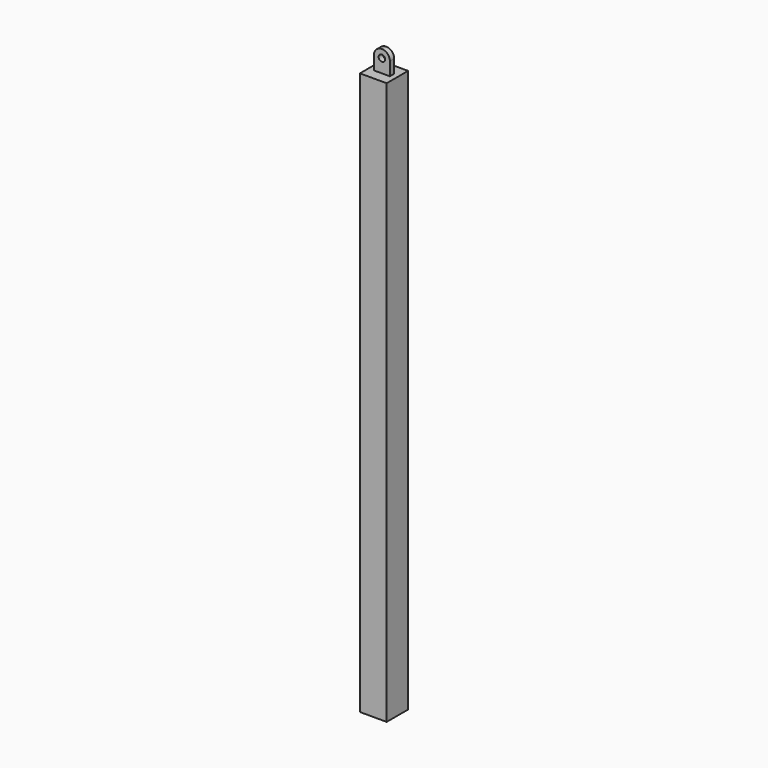
from build123d import *

# Parameters (mm, degrees)
F0_W     = 31.75
F0_H     = 666.75
F1_DEPTH = 31.75
F2_W     = 19.05
F2_H     = 6.35
F3_DEPTH = 25.4
F4_R     = 9.52499
F5_R     = 3.81
F6_DEPTH = 6.35
F7_W     = 1.5875
F7_H     = 12.7
F8_DEPTH = 22.225


# Not quite as in the source:
# - a fillet or chamfer is up to 0.001 mm smaller than in the source, because OpenCascade refuses the exact size


with BuildPart() as f1:
    # F0 (on Front) → F1 (new body)
    with BuildSketch(Plane.XZ):
        with Locations((-15.875, 127.5886728781)):
            Rectangle(F0_W, F0_H)
    extrude(amount=-F1_DEPTH)

    # F2 (on face) → F3 (join)
    with BuildSketch(Plane.XY.offset(460.9636728781)):
        with Locations((-15.875, 15.875)):
            Rectangle(F2_W, F2_H)
    extrude(amount=F3_DEPTH)

    # F4 (radius 9.525 in the source; OpenCascade refuses exactly that, so slightly less here)
    f4_edges = [f1.edges().sort_by_distance(p)[0] for p in [
        (-6.35, 15.875, 486.363673),
        (-25.4, 15.875, 486.363673),
    ]]
    fillet(f4_edges, radius=F4_R)

    # F5 (on face) → F6 (cut)
    with BuildSketch(Plane.XZ.offset(-12.7)):
        with Locations((-15.875, 476.8386728781)):
            Circle(F5_R)
    extrude(amount=-F6_DEPTH, mode=Mode.SUBTRACT)

    # F7 (on face) → F8 (cut)
    with BuildSketch(Plane(origin=(-31.75, 0, 0), x_dir=(0, -1, 0), z_dir=(-1, 0, 0))):
        with Locations((-29.36875, -177.2113271219)):
            Rectangle(F7_W, F7_H)
    extrude(amount=-F8_DEPTH, mode=Mode.SUBTRACT)


solid = f1.part
